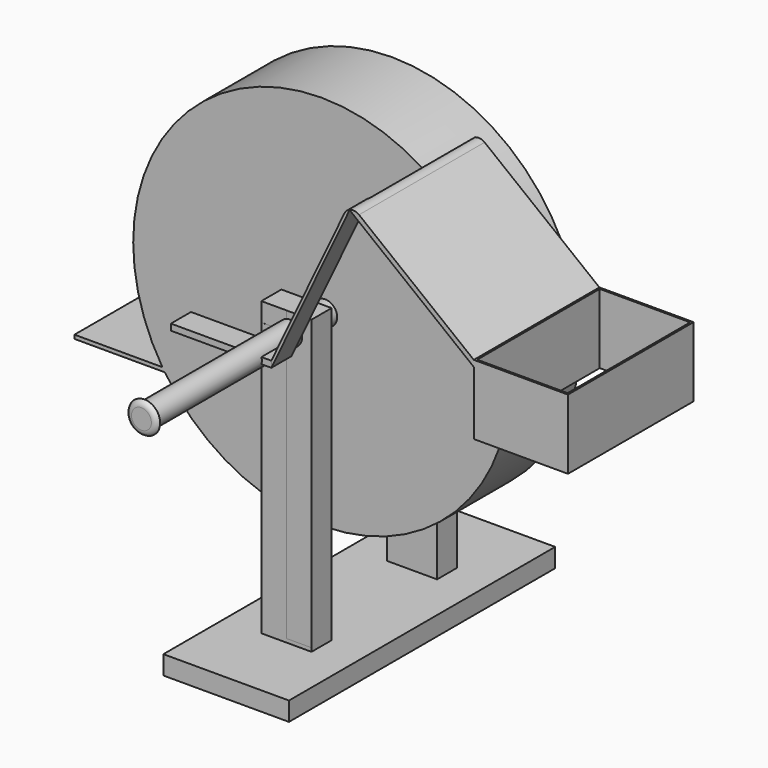
from build123d import *

# Parameters (mm, degrees)
F0_R         = 150
F1_DEPTH     = 70
F2_W         = 70
F2_H         = 3
F3_DEPTH     = 196.784
F5_R         = 9.5
F6_DEPTH     = 180
F7_R         = 9.5
F8_DEPTH     = 40
F9_W         = 20
F9_H         = 215
F10_DEPTH    = 20
F11_W        = 20
F11_H        = 18.9998925924
F11_H_2      = 196.0001074076
F12_DEPTH    = 20
F13_W        = 20
F13_H        = 20
F14_DEPTH    = 15
F15_W        = 40
F15_H        = 20
F16_DEPTH    = 25
F17_W        = 20
F17_H        = 215
F17_H_2      = 15
F18_DEPTH    = 20
F19_W        = 20
F19_H        = 20
F20_DEPTH    = 15
F21_W        = 20
F21_H        = 20
F22_DEPTH    = 215
F23_W        = 40
F23_H        = 19.9821153283
F24_DEPTH    = 15.5
F26_DEPTH    = 50
F28_DEPTH    = 50
F30_DEPTH    = 60
F31_DEPTH    = 20
F34_DEPTH    = 20
F36_DEPTH    = 125
F37_DEPTH    = 105
F38_W        = 72
F38_H        = 122
F30_FACE_W   = 53.7910459743
F30_FACE_H   = 20
F39_DEPTH    = 161
F40_R        = 12.5
F41_DEPTH    = 3
F43_R        = 9.5
F44_DEPTH    = 1
F45_T1_DEPTH = 172.813612667


# Not quite as in the source:
# - a fillet or chamfer that OpenCascade refuses, or shapes differently, is made with other operations: its cross-section is extruded or revolved along the edge and cut away or added


with BuildPart() as f1:
    # F0 (on Front) → F1 (new body)
    with BuildSketch(Plane.XZ):
        with Locations((0, -0.0713349276)):
            Circle(F0_R)
    extrude(amount=F1_DEPTH)

    # F2 (on Right) → F3 (join)
    with BuildSketch(Plane.YZ):
        with Locations((-35, -81.7328423858)):
            Rectangle(F2_W, F2_H)
    extrude(amount=-F3_DEPTH)

    # F5 (on face) → F6 (join)
    with BuildSketch(Plane.XZ.offset(70)):
        with Locations((2.9561973643, 0)):
            Circle(F5_R)
    extrude(amount=F6_DEPTH)

    # F7 (on face) → F8 (join)
    with BuildSketch(Plane(origin=(0, 0, 0), x_dir=(-1, 0, 0), z_dir=(0, 1, 0))):
        Circle(F7_R)
    extrude(amount=F8_DEPTH)

    # F9 (on Right) → F10 (join)
    with BuildSketch(Plane.YZ):
        with Locations((30, -98.0001074076)):
            Rectangle(F9_W, F9_H)
    extrude(amount=-F10_DEPTH)

    # F11 (on face) → F12 (join)
    with BuildSketch(Plane.YZ):
        with Locations((30, -5.37038e-05)):
            Rectangle(F11_W, F11_H)
        with Locations((30, -107.5000537038)):
            Rectangle(F11_W, F11_H_2)
    extrude(amount=F12_DEPTH)

    # F13 (on Top) → F14 (join)
    with BuildSketch(Plane.XY):
        with Locations((-10, 30)):
            Rectangle(F13_W, F13_H)
        with Locations((10, 30)):
            Rectangle(F13_W, F13_H)
    extrude(amount=F14_DEPTH)

    # F15 (on face) → F16 (join)
    with BuildSketch(Plane(origin=(0, 0, -205.5001074076), x_dir=(1, 0, 0), z_dir=(0, 0, -1))):
        with Locations((0, -30)):
            Rectangle(F15_W, F15_H)
    extrude(amount=F16_DEPTH)

    # F17 (on Right) → F18 (join)
    with BuildSketch(Plane.YZ):
        with Locations((-95, -107.5)):
            Rectangle(F17_W, F17_H)
        with Locations((-95, 7.5)):
            Rectangle(F17_W, F17_H_2)
    extrude(amount=F18_DEPTH)

    # F19 (on Top) → F20 (join)
    with BuildSketch(Plane.XY):
        with Locations((-10, -94.9609184265)):
            Rectangle(F19_W, F19_H)
    extrude(amount=F20_DEPTH)

    # F21 (on Top) → F22 (join)
    with BuildSketch(Plane.XY):
        with Locations((-10, -94.9821153283)):
            Rectangle(F21_W, F21_H)
    extrude(amount=-F22_DEPTH)

    # F23 (on face) → F24 (join)
    with BuildSketch(Plane(origin=(0, 0, -215), x_dir=(1, 0, 0), z_dir=(0, 0, -1))):
        with Locations((0, 94.9910576642)):
            Rectangle(F23_W, F23_H)
    extrude(amount=F24_DEPTH)

    # F25 (on Right) → F26 (join)
    with BuildSketch(Plane.YZ):
        Polygon((40.000025183, -230.4975450993), (40.0528562069, -217.8975450993), (40.0000102818, -217.8975450993), (-141.9770932198, -217.8975450993), (-164.9471437931, -217.8975450993), (-164.9471437931, -232.8975450993), (-126.0763406754, -232.8975450993), (20.0036764145, -232.8975450993), (40.000025183, -232.8975450993), align=None)
        Polygon((100.0528562069, -217.8975450993), (40.0528562069, -217.8975450993), (40.000025183, -230.4975450993), (40.000025183, -232.8975450993), (100.0528562069, -232.8975450993), align=None)
    extrude(amount=F26_DEPTH)

    # F27 (on face) → F28 (join)
    with BuildSketch(Plane(origin=(0, 0, 0), x_dir=(0, -1, 0), z_dir=(-1, 0, 0))):
        Polygon((164.9471437931, -217.8975450993), (-100.0528562069, -217.8975450993), (-100.0528562069, -232.8975450993), (-40, -232.8975450993), (164.9471437931, -232.8975450993), align=None)
    extrude(amount=F28_DEPTH)

    # F29 (on Right) → F30 (join)
    with BuildSketch(Plane.YZ):
        Polygon((-145, 2.5), (-145, -2.5), (-125, -2.5), (-125, 0), (-125, 2.5), align=None)
    extrude(amount=-F30_DEPTH)

    # F29 (on Right) → F31 (join)
    with BuildSketch(Plane.YZ):
        Polygon((-145, 2.5), (-145, -2.5), (-125, -2.5), (-125, 0), (-125, 2.5), align=None)
    extrude(amount=F31_DEPTH)

    # F40 (on face) → F41 (join)
    with BuildSketch(Plane.XZ.offset(250)):
        with Locations((2.9561973643, 0)):
            Circle(F40_R)
    extrude(amount=F41_DEPTH)

    # F42: fillet of radius 5 on 1 edges, made by hand

    # F42_s1 → F42_t2 (revolve, cut)
    with BuildSketch(Plane.XY):
        with BuildLine():
            ThreePointArc((15.4561973643, -250), (13.6122344568, -252.1833001327), (10.8736216693, -253))
            Line((10.8736216693, -253), (15.4561973643, -253))
            Line((15.4561973643, -253), (15.4561973643, -250))
        make_face()
    revolve(axis=Axis((2.9561973643, -253, 0), (0, -1, 0)), mode=Mode.SUBTRACT)

    # F43 (on face) → F44 (join)
    with BuildSketch(Plane(origin=(0, 40, 0), x_dir=(-1, 0, 0), z_dir=(0, 1, 0))):
        Circle(F43_R)
    extrude(amount=F44_DEPTH)


with BuildPart() as f34:
    # F33 (on offset) → F34 (new body)
    with BuildSketch(Plane(origin=(0, -125, 0), x_dir=(-1, 0, 0), z_dir=(0, 1, 0))):
        Polygon((-20.0000386685, -2.5), (-20.0000386685, 0), (-20.0000386685, 2.5), (-82.3409290722, 133.4145270154), (-181.2517998233, 55.5228017236), (-181.2517998233, 50.5228017236), (-82.3409290722, 128.4145270154), align=None)
        Polygon((-181.2517998233, 50.5228017236), (-181.2517998233, 55.5228017236), (-256.2517998233, 55.5228017236), (-256.2517998233, 0), (-181.2517998233, 0), align=None)
    extrude(amount=-F34_DEPTH)

    # F35 (on face) → F36 (join)
    with BuildSketch(Plane.XZ.offset(145)):
        Polygon((80.6093108737, 129.7781660978), (82.3409290722, 128.4145270154), (181.2517998233, 50.5228017236), (181.2517998233, 55.5228017236), (82.3409290722, 133.4145270154), align=None)
    extrude(amount=-F36_DEPTH)

    # F37 (add): a face of the model
    f37_faces = [f34.faces().sort_by_distance(p)[0] for p in [
        (218.7517998233, -125, 27.7614008618),
    ]]
    extrude(f37_faces, amount=F37_DEPTH)

    # F38 (on face) + F30_face (on face) → F39 (cut)
    with BuildSketch(Plane.XY.offset(55.5228017236)):
        with Locations((218.7517998233, -82.5)):
            Rectangle(F38_W, F38_H)
    with BuildSketch(Plane(origin=(-33.1044770128, -135, 2.5), x_dir=(1, 0, 0), z_dir=(0, 0, 1))):
        Rectangle(F30_FACE_W, F30_FACE_H)
    extrude(amount=-F39_DEPTH, mode=Mode.SUBTRACT)

    # F45: fillet of radius 7.6397458968 on 1 edges, made by hand

    # F45_s2 → F45_t1 (cut)
    with BuildSketch(Plane.XZ.offset(-3.9068063335)):
        with BuildLine():
            ThreePointArc((78.229559159, 124.7807387572), (83.3880678847, 128.9352971366), (89.8537727751, 127.4982070657))
            Line((89.8537727751, 127.4982070657), (82.3409290722, 133.4145270154))
            Line((82.3409290722, 133.4145270154), (78.229559159, 124.7807387572))
        make_face()
    extrude(amount=F45_T1_DEPTH, mode=Mode.SUBTRACT)


solid = Compound([f1.part, f34.part])
